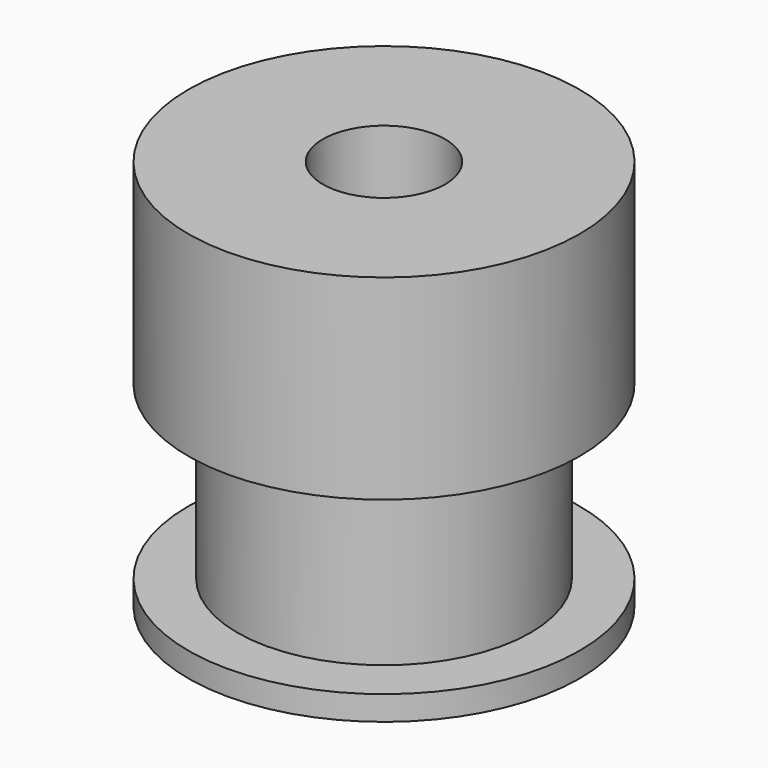
from build123d import *

# Parameters (mm, degrees)
F0_R     = 8
F0_R_2   = 6
F1_DEPTH = 8
F2_DEPTH = 7
F3_R     = 8
F3_R_2   = 6
F3_R_3   = 2.5
F4_DEPTH = 1
F5_DEPTH = 15.001


# Not quite as in the source:
# - a feature names something its author has since deleted; it is built from what else it names


with BuildPart() as f1:
    # F0 (on Top) → F1 (new body)
    with BuildSketch(Plane.XY):
        Circle(F0_R)
        Circle(F0_R_2, mode=Mode.SUBTRACT)
        Circle(F0_R_2)
    extrude(amount=F1_DEPTH)

    # F0 (on Top) → F2 (join)
    with BuildSketch(Plane.XY):
        Circle(F0_R_2)
    extrude(amount=-F2_DEPTH)

    # F3 (on face) → F4 (join)
    with BuildSketch(Plane(origin=(0, 0, -7), x_dir=(1, 0, 0), z_dir=(0, 0, -1))):
        Circle(F3_R)
        Circle(F3_R_2, mode=Mode.SUBTRACT)
        Circle(F3_R_2)
        Circle(F3_R_3, mode=Mode.SUBTRACT)
    extrude(amount=F4_DEPTH)

    # F3 (on face) → F5 (cut, through all)
    with BuildSketch(Plane(origin=(0, 0, -7), x_dir=(1, 0, 0), z_dir=(0, 0, -1))):
        Circle(F3_R_3)
    extrude(amount=-F5_DEPTH, mode=Mode.SUBTRACT)


solid = f1.part
